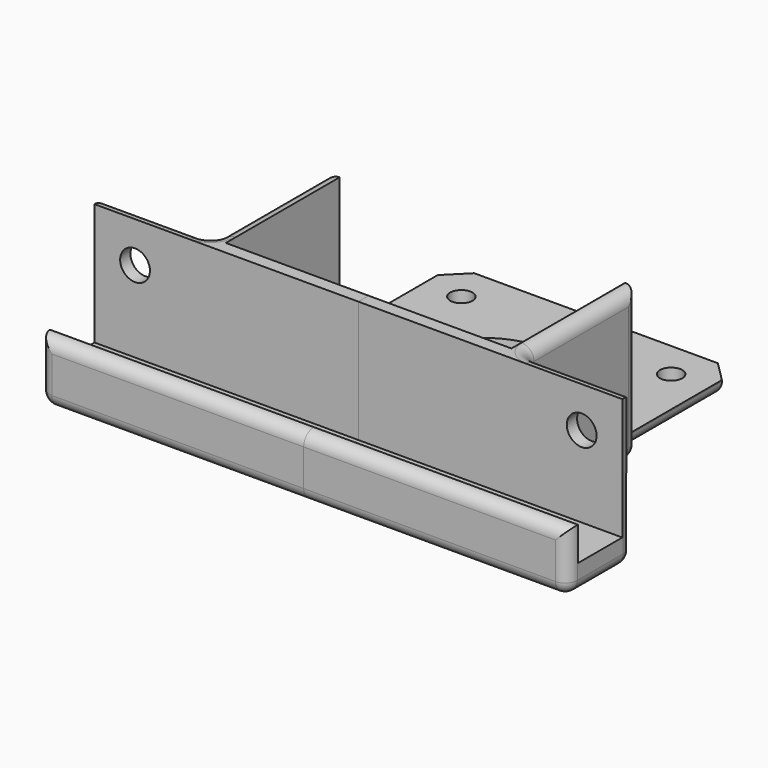
from build123d import *
from build123d import SkipClean  # not in build123d's __all__

# Parameters (mm, degrees)
F1_DEPTH  = 2
F3_DEPTH  = 2
F5_DEPTH  = 18
F6_W      = 39
F6_H      = 1.9
F7_DEPTH  = 5
F9_D      = 3.3
F9_DEPTH  = 8
F9_TIP    = 0.9914200214
F11_D     = 4.4
F11_DEPTH = 8
F11_TIP   = 1.3218933619
F12_R     = 1.8


with BuildPart() as f1:
    # F0 (on Top) → F1 (new body)
    with BuildSketch(Plane.XY):
        with BuildLine():
            Line((0, 21.5), (0, 0))
            Line((0, 0), (39, 0))
            Line((39, 0), (39, 12))
            Line((39, 12), (23, 12))
            Line((23, 12), (23, 33))
            Line((23, 33), (21, 33))
            Line((21, 33), (21, 51))
            Line((21, 51), (18, 54))
            Line((18, 54), (0, 54))
            Line((0, 54), (0, 44.5))
            ThreePointArc((0, 44.5), (11.5, 33), (0, 21.5))
        make_face()
    extrude(amount=F1_DEPTH)

    # F2 (on face) → F3 (join)
    with BuildSketch(Plane.XY.offset(2)):
        Polygon((0, 12), (0, 0), (39, 0), (39, 12), (23, 12), (23, 33), (21.1, 33), (21.1, 12), align=None)
    extrude(amount=F3_DEPTH)

    # F4 (on face) → F5 (join)
    with BuildSketch(Plane.XY.offset(4)):
        Polygon((23, 33), (21.1, 33), (21.1, 12), (0, 12), (0, 10.1), (39, 10.1), (39, 12), (23, 12), align=None)
    extrude(amount=F5_DEPTH)

    # F6 (on face) → F7 (join)
    with BuildSketch(Plane.XY.offset(4)):
        with Locations((19.5, 0.95)):
            Rectangle(F6_W, F6_H)
    extrude(amount=F7_DEPTH)

    # F9
    with Locations(Plane(origin=(0, 0, 0), x_dir=(1, 0, 0), z_dir=(0, 0, -1))):
        with Locations((15.5, -17.5), (15.5, -48.5)):
            Hole(F9_D / 2, depth=F9_DEPTH)
            with Locations((0, 0, -(F9_DEPTH + F9_TIP / 2))):  # 118° drill point
                Cone(0, F9_D / 2, F9_TIP, mode=Mode.SUBTRACT)

    # F11
    with Locations(Plane.XZ.offset(-10.1)):
        with Locations((33, 16)):
            Hole(F11_D / 2, depth=F11_DEPTH)
            with Locations((0, 0, -(F11_DEPTH + F11_TIP / 2))):  # 118° drill point
                Cone(0, F11_D / 2, F11_TIP, mode=Mode.SUBTRACT)

    # F12
    f12_edges = [f1.edges().sort_by_distance(p)[0] for p in [
        (31, 12, 22),
        (39, 12, 11),
        (23, 33, 11),
        (23, 22.5, 22),
        (23, 22.5, 0),
        (9, 54, 0),
        (31, 12, 0),
        (23, 12, 11),
        (39, 6, 0),
        (19.5, 0, 9),
        (19.5, 0, 0),
        (39, 0, 4.5),
        (21, 42, 0),
        (22, 33, 0),
        (19.5, 52.5, 0),
    ]]
    fillet(f12_edges, radius=F12_R)

    # F13: F1 across plane


with BuildPart() as f1_1:
    add(f1.part, clean=False)
    with SkipClean():  # cleaning this boolean's faces spoils the solid; the shape is the same uncleaned
        add(f1.part.mirror(Plane.YZ), clean=False)


solid = f1_1.part
